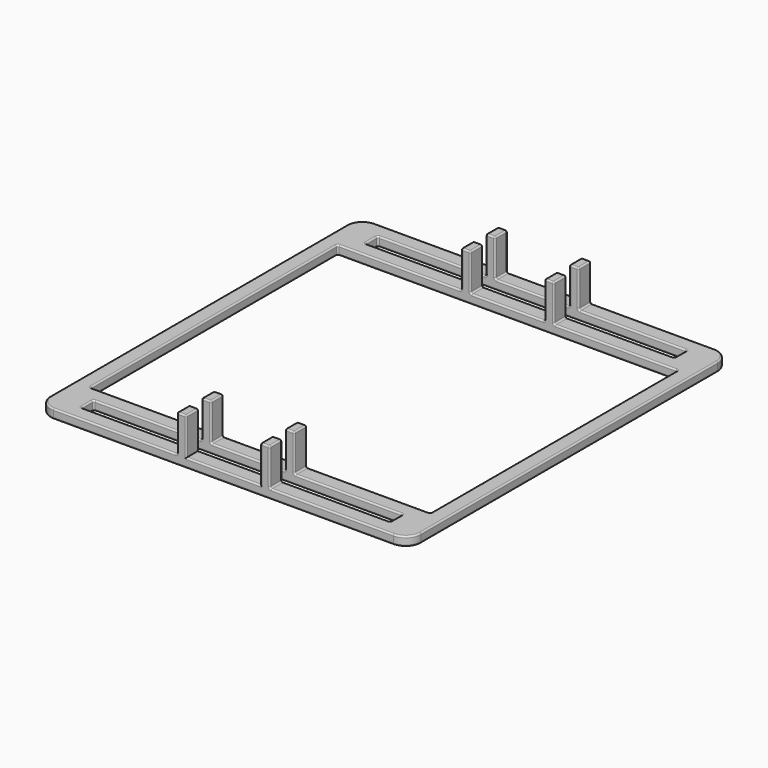
from build123d import *

# Parameters (mm, degrees)
F1_DEPTH = 3
F0_W     = 3
F0_H     = 5
F2_DEPTH = 15
F0_W_2   = 24
F3_DEPTH = 3
F5_R     = 5
F6_F1_R  = 0.5
F6_F2_R  = 0.5


with BuildPart() as f1:
    # F0 (on Top) → F1 (new body)
    with BuildSketch(Plane.XY):
        Polygon((-15, 55), (-50, 55), (-50, 60), (-15, 60), (-15, 65), (-55, 65), (-60, 65), (-60, 60), (-60, 55), (-60, -55), (-60, -60), (-60, -65), (-55, -65), (-15, -65), (-15, -60), (-50, -60), (-50, -55), (-15, -55), (-15, -50), (-55, -50), (-55, 50), (-15, 50), align=None)
    extrude(amount=F1_DEPTH)


with BuildPart() as f1b:
    # F0 (on Top) → F1, piece 2 (new body)
    with BuildSketch(Plane.XY):
        Polygon((50, 55), (15, 55), (15, 50), (55, 50), (55, -50), (15, -50), (15, -55), (50, -55), (50, -60), (15, -60), (15, -65), (55, -65), (60, -65), (60, -60), (60, -55), (60, 55), (60, 60), (60, 65), (55, 65), (15, 65), (15, 60), (50, 60), align=None)
    extrude(amount=F1_DEPTH)


with BuildPart() as f2:
    # F0 (on Top) → F2 (new body)
    with BuildSketch(Plane.XY):
        with Locations((-13.5, 62.5)):
            Rectangle(F0_W, F0_H)
    extrude(amount=F2_DEPTH)


with BuildPart() as f2b:
    # F0 (on Top) → F2, piece 2 (new body)
    with BuildSketch(Plane.XY):
        with Locations((-13.5, 52.5)):
            Rectangle(F0_W, F0_H)
    extrude(amount=F2_DEPTH)


with BuildPart() as f2c:
    # F0 (on Top) → F2, piece 3 (new body)
    with BuildSketch(Plane.XY):
        with Locations((13.5, 52.5)):
            Rectangle(F0_W, F0_H)
    extrude(amount=F2_DEPTH)


with BuildPart() as f2d:
    # F0 (on Top) → F2, piece 4 (new body)
    with BuildSketch(Plane.XY):
        with Locations((13.5, 62.5)):
            Rectangle(F0_W, F0_H)
    extrude(amount=F2_DEPTH)


with BuildPart() as f2e:
    # F0 (on Top) → F2, piece 5 (new body)
    with BuildSketch(Plane.XY):
        with Locations((13.5, -52.5)):
            Rectangle(F0_W, F0_H)
    extrude(amount=F2_DEPTH)


with BuildPart() as f2f:
    # F0 (on Top) → F2, piece 6 (new body)
    with BuildSketch(Plane.XY):
        with Locations((13.5, -62.5)):
            Rectangle(F0_W, F0_H)
    extrude(amount=F2_DEPTH)


with BuildPart() as f2g:
    # F0 (on Top) → F2, piece 7 (new body)
    with BuildSketch(Plane.XY):
        with Locations((-13.5, -62.5)):
            Rectangle(F0_W, F0_H)
    extrude(amount=F2_DEPTH)


with BuildPart() as f2h:
    # F0 (on Top) → F2, piece 8 (new body)
    with BuildSketch(Plane.XY):
        with Locations((-13.5, -52.5)):
            Rectangle(F0_W, F0_H)
    extrude(amount=F2_DEPTH)


with BuildPart() as f3:
    # F0 (on Top) → F3 (new body)
    with BuildSketch(Plane.XY):
        with Locations((0, 62.5)):
            Rectangle(F0_W_2, F0_H)
    extrude(amount=F3_DEPTH)


with BuildPart() as f3b:
    # F0 (on Top) → F3, piece 2 (new body)
    with BuildSketch(Plane.XY):
        with Locations((0, 52.5)):
            Rectangle(F0_W_2, F0_H)
    extrude(amount=F3_DEPTH)


with BuildPart() as f3c:
    # F0 (on Top) → F3, piece 3 (new body)
    with BuildSketch(Plane.XY):
        with Locations((0, -52.5)):
            Rectangle(F0_W_2, F0_H)
    extrude(amount=F3_DEPTH)


with BuildPart() as f3d:
    # F0 (on Top) → F3, piece 4 (new body)
    with BuildSketch(Plane.XY):
        with Locations((0, -62.5)):
            Rectangle(F0_W_2, F0_H)
    extrude(amount=F3_DEPTH)


with BuildPart() as f1_1:
    add(f1.part)

    # F4: union F1b, F2c, F2d, F2h, F2e, F2g, F2f, F2b, F2, F3b, F3, F3c, F3d
    add(f1b.part)
    add(f2c.part)
    add(f2d.part)
    add(f2h.part)
    add(f2e.part)
    add(f2g.part)
    add(f2f.part)
    add(f2b.part)
    add(f2.part)
    add(f3b.part)
    add(f3.part)
    add(f3c.part)
    add(f3d.part)

    # F5
    f5_edges = [f1_1.edges().sort_by_distance(p)[0] for p in [
        (60, -65, 1.5),
        (60, 65, 1.5),
        (-60, -65, 1.5),
        (-60, 65, 1.5),
    ]]
    fillet(f5_edges, radius=F5_R)

    # F6: fillet of radius 0.5 on 131 edges, made by hand

    # F6_f1
    f6_f1_edges = [f1_1.edges().sort_by_distance(p)[0] for p in [
        (-15, 62.5, 3),
        (-15, -62.5, 3),
        (-15, 52.5, 3),
        (-15, -52.5, 3),
        (15, -62.5, 3),
        (15, 62.5, 3),
        (15, -52.5, 3),
        (15, 52.5, 3),
        (-50, -55, 1.5),
        (50, -55, 1.5),
        (-50, -60, 1.5),
        (50, -60, 1.5),
        (-55, 50, 1.5),
        (55, 50, 1.5),
        (-50, 60, 1.5),
        (50, 60, 1.5),
        (-50, 55, 1.5),
        (50, 55, 1.5),
        (-12, 62.5, 3),
        (12, 62.5, 3),
        (-12, 52.5, 3),
        (12, 52.5, 3),
        (-12, -52.5, 3),
        (12, -52.5, 3),
        (-55, -50, 1.5),
        (55, -50, 1.5),
    ]]
    fillet(f6_f1_edges, radius=F6_F1_R)

    # F6_f2
    f6_f2_edges = [f1_1.edges().sort_by_distance(p)[0] for p in [
        (-35.25, 65, 3),
        (-58.5355339059, 63.5355339059, 3),
        (-60, 0, 3),
        (-32.5, 60, 3),
        (-58.5355339059, -63.5355339059, 3),
        (-50, 57.5, 3),
        (-35.25, -65, 3),
        (-32.5, 55, 3),
        (-32.5, -60, 3),
        (-35, 50, 3),
        (-50, -57.5, 3),
        (-55, 0, 3),
        (-32.5, -55, 3),
        (-35, -50, 3),
        (35.25, -65, 3),
        (58.5355339059, -63.5355339059, 3),
        (60, 0, 3),
        (32.5, -60, 3),
        (58.5355339059, 63.5355339059, 3),
        (50, -57.5, 3),
        (35.25, 65, 3),
        (32.5, -55, 3),
        (32.5, 60, 3),
        (35, -50, 3),
        (50, 57.5, 3),
        (55, 0, 3),
        (32.5, 55, 3),
        (35, 50, 3),
        (-15, -65, 9.25),
        (0, -65, 0),
        (-13.5, -65, 15),
        (-12, -65, 9),
        (0, -65, 3),
        (15, -65, 9.25),
        (12, -65, 9),
        (13.5, -65, 15),
        (-15, -55, 9.25),
        (-13.5, -55, 15),
        (-12, -55, 9.25),
        (0, -55, 3),
        (12, -55, 9.25),
        (13.5, -55, 15),
        (15, -55, 9.25),
        (0, -55, 0),
        (0, -60, 0),
        (15, -60, 9.25),
        (13.5, -60, 15),
        (12, -60, 9),
        (0, -60, 3),
        (-12, -60, 9),
        (-13.5, -60, 15),
        (-15, -60, 9.25),
        (-15, 50, 9.25),
        (-13.5, 50, 15),
        (-12, 50, 9.25),
        (0, 50, 3),
        (12, 50, 9.25),
        (13.5, 50, 15),
        (15, 50, 9.25),
        (0, 50, 0),
        (-15, 60, 9.25),
        (-13.5, 60, 15),
        (-12, 60, 9.25),
        (0, 60, 3),
        (12, 60, 9.25),
        (13.5, 60, 15),
        (15, 60, 9.25),
        (0, 60, 0),
        (0, 55, 0),
        (15, 55, 9.25),
        (13.5, 55, 15),
        (12, 55, 9.25),
        (0, 55, 3),
        (-12, 55, 9.25),
        (-13.5, 55, 15),
        (-15, 55, 9.25),
        (0, 65, 3),
        (0, -50, 3),
        (0, -50, 0),
        (15, -50, 9.25),
        (13.5, -50, 15),
        (12, -50, 9.25),
        (-12, -50, 9.25),
        (-13.5, -50, 15),
        (-15, -50, 9.25),
        (12, -52.5, 15),
        (15, -52.5, 15),
        (12, -62.5, 15),
        (15, -62.5, 15),
        (-15, -62.5, 15),
        (-12, -62.5, 15),
        (-15, -52.5, 15),
        (-12, -52.5, 15),
        (-15, 62.5, 15),
        (-12, 62.5, 15),
        (-13.5, 65, 15),
        (-15, 52.5, 15),
        (-12, 52.5, 15),
        (12, 52.5, 15),
        (15, 52.5, 15),
        (12, 62.5, 15),
        (15, 62.5, 15),
        (13.5, 65, 15),
        (58.5355339059, -63.5355339059, 0),
        (-58.5355339059, -63.5355339059, 0),
        (-60, 0, 0),
        (-58.5355339059, 63.5355339059, 0),
        (0, 65, 0),
        (58.5355339059, 63.5355339059, 0),
        (60, 0, 0),
        (-15.1464466094, -50, 3.1464466094),
        (-11.8535533906, -50, 3.1464466094),
        (11.8535533906, -50, 3.1464466094),
        (15.1464466094, -50, 3.1464466094),
        (-54.8535533906, -49.8535533906, 0),
        (54.8535533906, -49.8535533906, 0),
        (11.8535533906, 65, 3.1464466094),
        (-11.8535533906, 65, 3.1464466094),
        (-15.1464466094, 55, 3.1464466094),
        (-11.8535533906, 55, 3.1464466094),
        (11.8535533906, 55, 3.1464466094),
        (15.1464466094, 55, 3.1464466094),
        (49.8535533906, 55.1464466094, 0),
        (-49.8535533906, 55.1464466094, 0),
        (49.8535533906, 59.8535533906, 0),
        (-49.8535533906, 59.8535533906, 0),
        (15.1464466094, 60, 3.1464466094),
        (11.8535533906, 60, 3.1464466094),
        (-11.8535533906, 60, 3.1464466094),
        (-15.1464466094, 60, 3.1464466094),
        (54.8535533906, 49.8535533906, 0),
        (-54.8535533906, 49.8535533906, 0),
        (15.1464466094, 50, 3.1464466094),
        (11.8535533906, 50, 3.1464466094),
        (-11.8535533906, 50, 3.1464466094),
        (-15.1464466094, 50, 3.1464466094),
        (-15.1464466094, -60, 3.1464466094),
        (15.1464466094, -60, 3.1464466094),
        (-49.8535533906, -59.8535533906, 0),
        (49.8535533906, -59.8535533906, 0),
        (49.8535533906, -55.1464466094, 0),
        (-49.8535533906, -55.1464466094, 0),
        (15.1464466094, -55, 3.1464466094),
        (11.8535533906, -55, 3.1464466094),
        (-11.8535533906, -55, 3.1464466094),
        (-15.1464466094, -55, 3.1464466094),
        (15.1464466094, -65, 3.1464466094),
        (-15.1464466094, -65, 3.1464466094),
        (54.8535533906, 49.8535533906, 3),
        (49.8535533906, 55.1464466094, 3),
        (54.8535533906, -49.8535533906, 3),
        (49.8535533906, 59.8535533906, 3),
        (49.8535533906, -55.1464466094, 3),
        (15.1464466094, 65, 3.1464466094),
        (49.8535533906, -59.8535533906, 3),
        (-54.8535533906, -49.8535533906, 3),
        (-49.8535533906, -55.1464466094, 3),
        (-54.8535533906, 49.8535533906, 3),
        (-49.8535533906, -59.8535533906, 3),
        (-49.8535533906, 55.1464466094, 3),
        (-49.8535533906, 59.8535533906, 3),
        (-15.1464466094, 65, 3.1464466094),
    ]]
    fillet(f6_f2_edges, radius=F6_F2_R)


solid = f1_1.part
